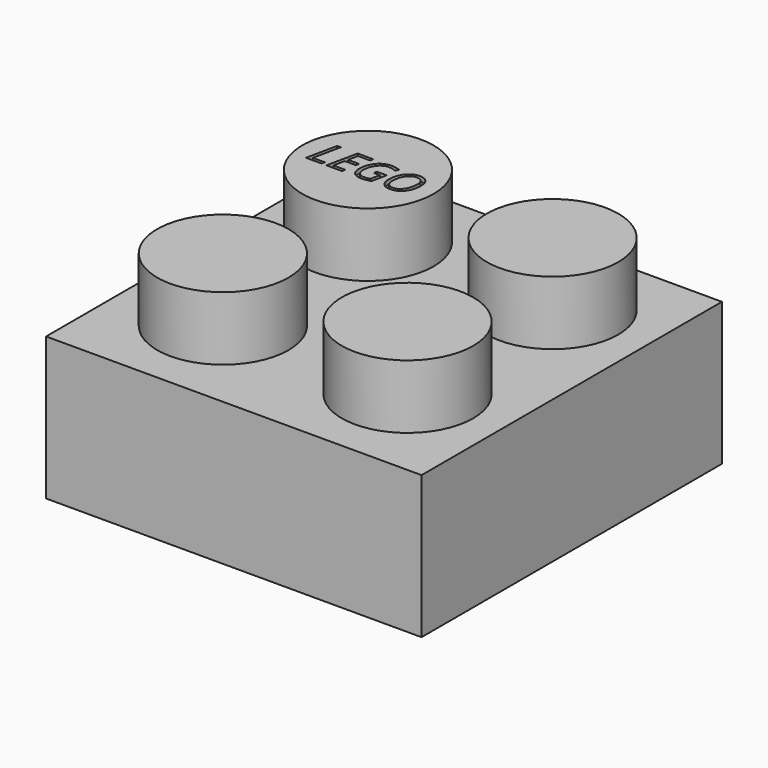
from build123d import *

# Parameters (mm, degrees)
F0_W         = 127
F0_H         = 127
F1_DEPTH     = 48.26
F2_R         = 22.225
F3_DEPTH     = 21.59
F4_TEXT_SIZE = 14.6249955934
F5_DEPTH     = 1.524


# Not quite as in the source:
# - Text() gives the source's letters only with a copy of the font that has no kerning and outlines rounded to 1/6400 em; it was checked with that copy


with BuildPart() as f1:
    # F0 (on Top) → F1 (new body)
    with BuildSketch(Plane.XY):
        Rectangle(F0_W, F0_H)
    extrude(amount=F1_DEPTH)

    # F2 (on face) → F3 (join)
    with BuildSketch(Plane.XY.offset(48.26)):
        with Locations((-30.8220349252, 31.7270830274)):
            Circle(F2_R)
        with Locations((31.6332392395, 31.7270830274)):
            Circle(F2_R)
        with Locations((31.6332392395, -29.6008400619)):
            Circle(F2_R)
        with Locations((-30.8220349252, -29.6008400619)):
            Circle(F2_R)
    extrude(amount=F3_DEPTH)

    # F4 (on face) → F5 (cut)
    with BuildSketch(Plane.XY.offset(69.85)):
        with Locations((-48.4502390027, 26.8086995929)):
            Text('LEGO', F4_TEXT_SIZE, font='Open Sans', font_style=FontStyle.ITALIC, text_align=(TextAlign.LEFT, TextAlign.BOTTOM))
    extrude(amount=-F5_DEPTH, mode=Mode.SUBTRACT)


solid = f1.part
